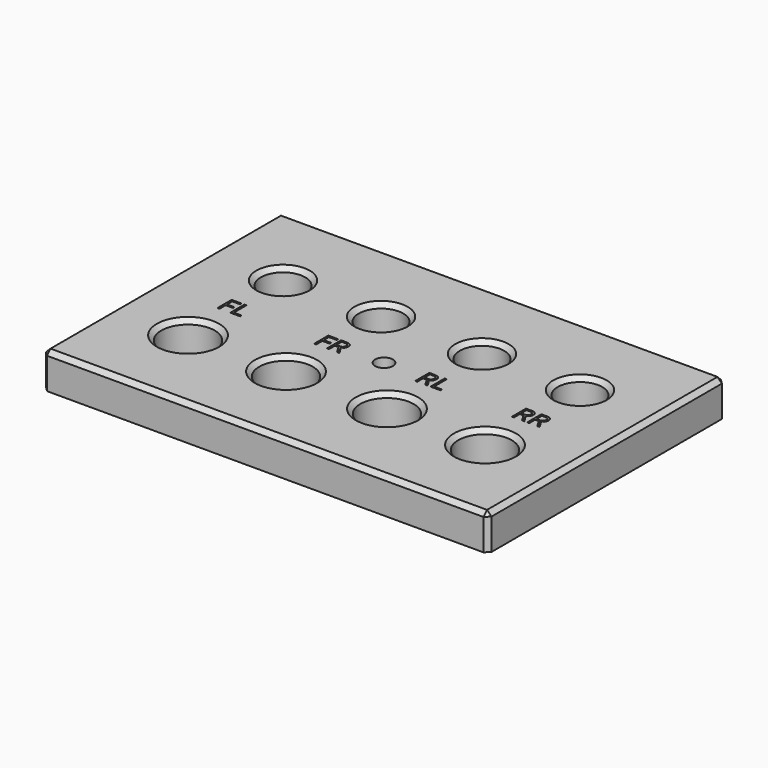
from build123d import *

# Parameters (mm, degrees)
F0_W           = 150
F0_H           = 100
F0_R           = 9
F0_R_2         = 7.5
F1_DEPTH       = 12
F2_SIZE        = 1.5
F3_SIZE        = 1.5
F4_D           = 3.4
F4_CBORE_D     = 6
F4_CBORE_DEPTH = 3.5
F5_TEXT_SIZE   = 8.3333333333
F6_DEPTH       = 1


# Not quite as in the source:
# - Text() gives the source's letters only with a copy of the font that has no kerning and outlines rounded to 1/6400 em; it was checked with that copy


with BuildPart() as f1:
    # F0 (on Top) → F1 (new body)
    with BuildSketch(Plane.XY):
        Rectangle(F0_W, F0_H)
        with Locations((-50, -20)):
            Circle(F0_R, mode=Mode.SUBTRACT)
        with Locations((-17, -20)):
            Circle(F0_R, mode=Mode.SUBTRACT)
        with Locations((17, -20)):
            Circle(F0_R, mode=Mode.SUBTRACT)
        with Locations((50, -20)):
            Circle(F0_R, mode=Mode.SUBTRACT)
        with Locations((-50, 20)):
            Circle(F0_R_2, mode=Mode.SUBTRACT)
        with Locations((-17, 20)):
            Circle(F0_R_2, mode=Mode.SUBTRACT)
        with Locations((17, 20)):
            Circle(F0_R_2, mode=Mode.SUBTRACT)
        with Locations((50, 20)):
            Circle(F0_R_2, mode=Mode.SUBTRACT)
    extrude(amount=-F1_DEPTH)

    # F2
    f2_edges = [f1.edges().sort_by_distance(p)[0] for p in [
        (-75, 50, -6),
        (75, 50, -6),
        (75, -50, -6),
        (-75, -50, -6),
        (0, 50, 0),
        (0, -50, 0),
        (-75, 0, 0),
        (75, 0, 0),
    ]]
    chamfer(f2_edges, length=F2_SIZE)

    # F3
    f3_edges = [f1.edges().sort_by_distance(p)[0] for p in [
        (-57.5, 20, 0),
        (-24.5, 20, 0),
        (9.5, 20, 0),
        (42.5, 20, 0),
        (-59, -20, 0),
        (-26, -20, 0),
        (8, -20, 0),
        (41, -20, 0),
    ]]
    chamfer(f3_edges, length=F3_SIZE)

    # F4 (through all)
    with Locations(Plane.XY):
        with Locations((0, 0)):
            CounterBoreHole(F4_D / 2, F4_CBORE_D / 2, F4_CBORE_DEPTH)

    # F5 (on Top) → F6 (cut)
    with BuildSketch(Plane.XY):
        with Locations((-54.4876302083, -3)):
            Text('FL', F5_TEXT_SIZE, font='Open Sans', text_align=(TextAlign.LEFT, TextAlign.BOTTOM))
        with Locations((-21.9251302083, -3)):
            Text('FR', F5_TEXT_SIZE, font='Open Sans', text_align=(TextAlign.LEFT, TextAlign.BOTTOM))
        with Locations((12.0872395833, -3)):
            Text('RL', F5_TEXT_SIZE, font='Open Sans', text_align=(TextAlign.LEFT, TextAlign.BOTTOM))
        with Locations((44.6497395833, -3)):
            Text('RR', F5_TEXT_SIZE, font='Open Sans', text_align=(TextAlign.LEFT, TextAlign.BOTTOM))
    extrude(amount=-F6_DEPTH, mode=Mode.SUBTRACT)


solid = f1.part
